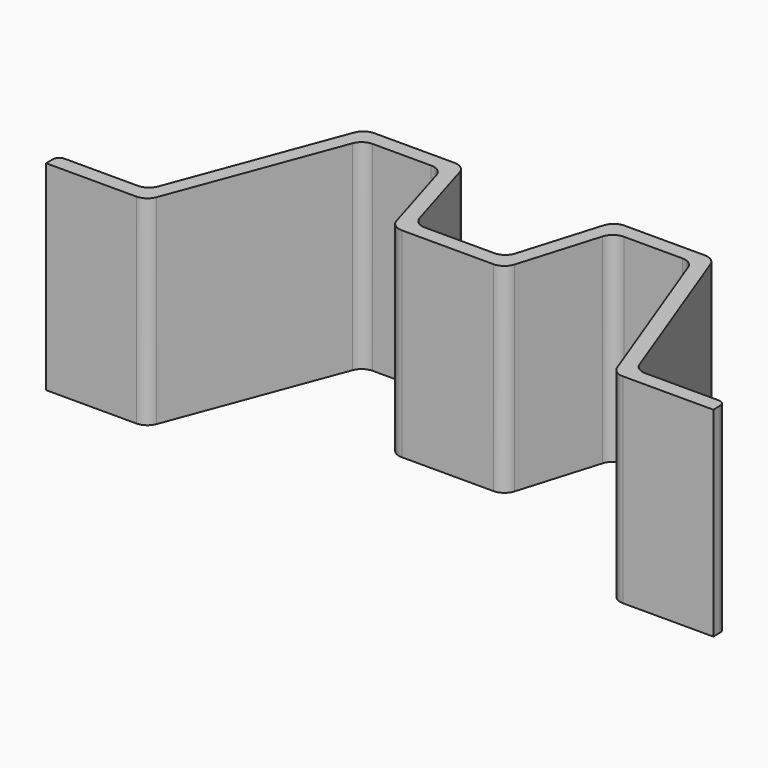
from build123d import *

# Parameters (mm, degrees)
F1_DEPTH = 20
F2_R     = 1.3846892623
F3_R     = 0.6428654195


# Not quite as in the source:
# - a feature names something its author has since deleted; it is built from what else it names


with BuildPart() as f1:
    # F0 (on Top) → F1 (new body)
    with BuildSketch(Plane.XY):
        Polygon((0, -1.5), (0, 0), (-4.5, 0), (-7.5, 10), (-17.5, 10), (-24.4375, -8.5), (-33.3979992978, -8.5), (-33.3979992978, -10), (-25, -10), (-23.3979992978, -10), (-16.4604992978, 8.5), (-8.6160459763, 8.5), (-5.6160459763, -1.5), align=None)
        Polygon((4.5, 0), (0, 0), (0, -1.5), (5.6160459763, -1.5), (8.6160459763, 8.5), (16.4604992978, 8.5), (23.3979992978, -10), (33.3979992978, -10), (33.3979992978, -8.5), (24.4375, -8.5), (17.5, 10), (7.5, 10), align=None)
    extrude(amount=F1_DEPTH)

    # F2
    f2_edges = [f1.edges().sort_by_distance(p)[0] for p in [
        (-7.5, 10, 10),
        (-4.5, 0, 10),
        (-17.5, 10, 10),
        (-16.460499, 8.5, 10),
        (-8.616046, 8.5, 10),
        (-5.616046, -1.5, 10),
        (17.5, 10, 10),
        (7.5, 10, 10),
        (4.5, 0, 10),
        (24.4375, -8.5, 10),
        (-24.4375, -8.5, 10),
        (5.616046, -1.5, 10),
        (8.616046, 8.5, 10),
        (16.460499, 8.5, 10),
        (23.397999, -10, 10),
        (-23.397999, -10, 10),
    ]]
    fillet(f2_edges, radius=F2_R)

    # F3
    f3_edges = [f1.edges().sort_by_distance(p)[0] for p in [
        (-33.397999, -8.5, 10),
        (33.397999, -8.5, 10),
    ]]
    fillet(f3_edges, radius=F3_R)


solid = f1.part
